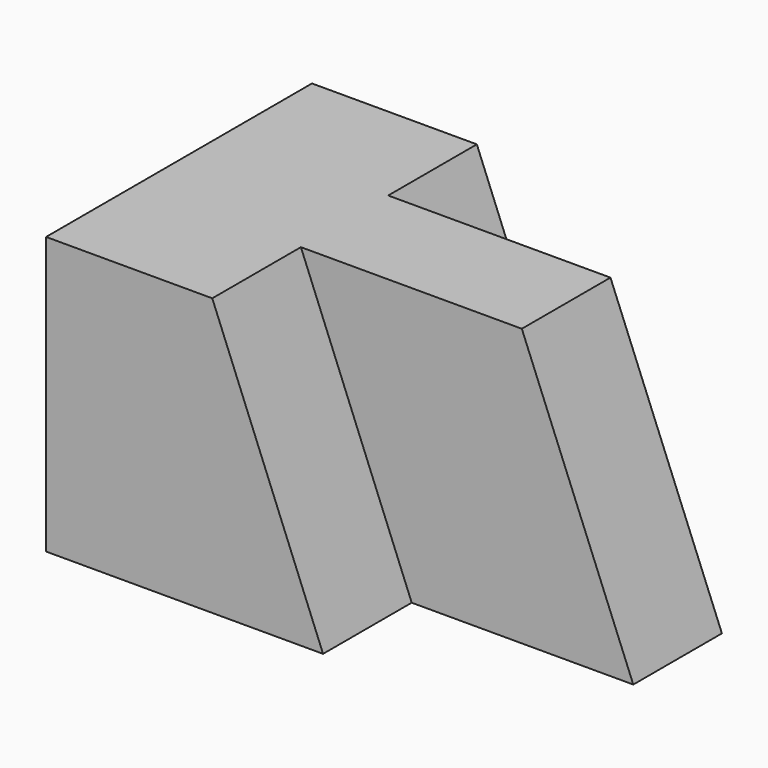
from build123d import *
from build123d import SkipClean  # not in build123d's __all__

# Parameters (mm, degrees)
F1_DEPTH = 31.75
F3_DEPTH = 12.7
F5_DEPTH = 12.7
F7_DEPTH = 25.401


with BuildPart() as f1:
    # F0 (on Top) → F1 (new body)
    with BuildSketch(Plane.XY):
        Polygon((31.597598396, 0), (0, -0.0003033445), (0, -38.1), (31.75, -38.1), (31.75, -25.4), (57.15, -25.4), (57.15, -12.7), (31.597598396, -12.7), align=None)
    extrude(amount=F1_DEPTH)

    # F2 (on face) → F3 (cut)
    with BuildSketch(Plane.XZ.offset(38.1)):
        Polygon((31.75, 0), (31.75, 31.75), (19.05, 31.75), align=None)
    extrude(amount=-F3_DEPTH, mode=Mode.SUBTRACT)

    # F4 (on face) → F5 (cut)
    with BuildSketch(Plane(origin=(2.9e-09, -0.0003033445, 0), x_dir=(-1, -9.6002e-06, 0), z_dir=(-9.6002e-06, 1, 0))):
        Polygon((-18.8975983945, 31.75), (-31.5975983945, 31.75), (-31.5975983945, 0), align=None)
    with SkipClean():  # cleaning this boolean's faces spoils the solid; the shape is the same uncleaned
        extrude(amount=-F5_DEPTH, mode=Mode.SUBTRACT)

    # F6 (on face) → F7 (cut, through all)
    with BuildSketch(Plane(origin=(0, -12.7, 0), x_dir=(-1, 0, 0), z_dir=(0, 1, 0))):
        Polygon((-44.373799198, 31.75), (-57.15, 31.75), (-57.15, 0), align=None)
    extrude(amount=-F7_DEPTH, mode=Mode.SUBTRACT)


solid = f1.part
